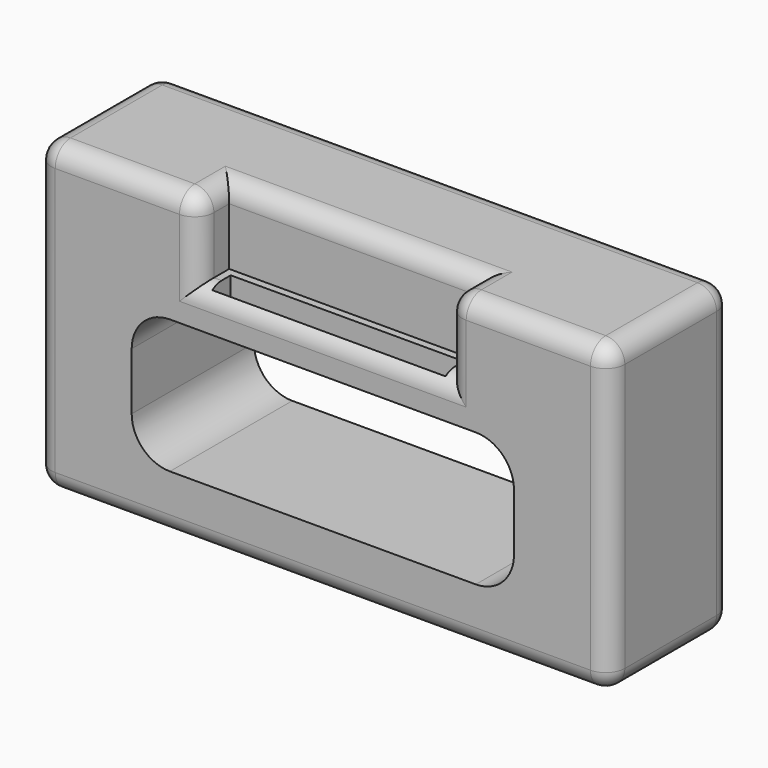
from build123d import *

# Parameters (mm, degrees)
F0_W          = 150
F0_H          = 40
F1_DEPTH      = 80
F2_W          = 65
F2_H          = 20
F3_DEPTH      = 10
F5_DEPTH      = 287
F6_W          = 61
F6_H          = 6
F7_DEPTH      = 25
F8_T1_DEPTH   = 65
F8_T3_DEPTH   = 70
F8_T5_DEPTH   = 32.5
F8_T7_DEPTH   = 32.5
F8_T9_DEPTH   = 30
F8_T11_DEPTH  = 140
F8_T13_DEPTH  = 15
F8_T15_DEPTH  = 5
F8_S19_W      = 5
F8_S19_H      = 5
F8_T20_DEPTH  = 5
F8_S25_W      = 5
F8_S25_H      = 5
F8_T26_DEPTH  = 5
F8_S31_W      = 5
F8_S31_H      = 5
F8_T32_DEPTH  = 5
F8_S37_W      = 5
F8_S37_H      = 5
F8_T38_DEPTH  = 5
F8_S43_W      = 5
F8_S43_H      = 5
F8_T44_DEPTH  = 5
F8_S49_W      = 5
F8_S49_H      = 5
F8_T50_DEPTH  = 5
F8_S55_W      = 5
F8_S55_H      = 5
F8_T56_DEPTH  = 5
F8_S61_W      = 5
F8_S61_H      = 5
F8_T62_DEPTH  = 5
F8_S67_W      = 5
F8_S67_H      = 5
F8_T68_DEPTH  = 5
F8_S73_W      = 5
F8_S73_H      = 5
F8_T74_DEPTH  = 5
F8_T81_DEPTH  = 17.5
F8_T85_DEPTH  = 77.5
F8_T92_DEPTH  = 77.5
F8_T96_DEPTH  = 17.5
F8_T103_DEPTH = 27.5
F8_T107_DEPTH = 77.5
F8_T114_DEPTH = 27.5
F8_T118_DEPTH = 77.5


# Not quite as in the source:
# - a fillet or chamfer that OpenCascade refuses, or shapes differently, is made with other operations: its cross-section is extruded or revolved along the edge and cut away or added


with BuildPart() as f1:
    # F0 (on Top) → F1 (new body)
    with BuildSketch(Plane.XY):
        with Locations((-14.0948228538, -1.1422424763)):
            Rectangle(F0_W, F0_H)
    extrude(amount=F1_DEPTH)

    # F2 (on face) → F3 (cut)
    with BuildSketch(Plane.XZ.offset(21.1422424763)):
        with Locations((-14.0948228538, 70)):
            Rectangle(F2_W, F2_H)
    extrude(amount=-F3_DEPTH, mode=Mode.SUBTRACT)

    # F4 (on face) → F5 (cut)
    with BuildSketch(Plane.XZ.offset(21.1422424763)):
        with BuildLine():
            Line((25.9051771462, 50), (-54.0948228538, 50))
            ThreePointArc((-54.0948228538, 50), (-61.1658906657, 47.0710678119), (-64.0948228538, 40))
            Line((-64.0948228538, 40), (-64.0948228538, 25))
            ThreePointArc((-64.0948228538, 25), (-61.1658906657, 17.9289321881), (-54.0948228538, 15))
            Line((-54.0948228538, 15), (25.9051771462, 15))
            ThreePointArc((25.9051771462, 15), (32.9762449581, 17.9289321881), (35.9051771462, 25))
            Line((35.9051771462, 25), (35.9051771462, 40))
            ThreePointArc((35.9051771462, 40), (32.9762449581, 47.0710678119), (25.9051771462, 50))
        make_face()
    extrude(amount=-F5_DEPTH, mode=Mode.SUBTRACT)

    # F6 (on face) → F7 (cut)
    with BuildSketch(Plane.XY.offset(60)):
        with Locations((-14.0948228538, -16.1422424763)):
            Rectangle(F6_W, F6_H)
    extrude(amount=-F7_DEPTH, mode=Mode.SUBTRACT)

    # F8: fillet of radius 5 on 19 edges, made by hand

    # F8_s2 → F8_t1 (cut)
    with BuildSketch(Plane.YZ.offset(-46.5948228538)):
        with BuildLine():
            ThreePointArc((-6.1422424763, 80), (-9.6777763823, 78.5355339059), (-11.1422424763, 75))
            Line((-11.1422424763, 75), (-11.1422424763, 80))
            Line((-11.1422424763, 80), (-6.1422424763, 80))
        make_face()
        with BuildLine():
            ThreePointArc((-21.1422424763, 55), (-19.6777763823, 58.5355339059), (-16.1422424763, 60))
            Line((-16.1422424763, 60), (-21.1422424763, 60))
            Line((-21.1422424763, 60), (-21.1422424763, 55))
        make_face()
    extrude(amount=F8_T1_DEPTH, mode=Mode.SUBTRACT)

    # F8_s4 → F8_t3 (cut)
    with BuildSketch(Plane.XY.offset(5)):
        with BuildLine():
            ThreePointArc((-84.0948228538, -21.1422424763), (-87.6303567597, -19.6777763823), (-89.0948228538, -16.1422424763))
            Line((-89.0948228538, -16.1422424763), (-89.0948228538, -21.1422424763))
            Line((-89.0948228538, -21.1422424763), (-84.0948228538, -21.1422424763))
        make_face()
        with BuildLine():
            ThreePointArc((60.9051771462, -16.1422424763), (59.4407110521, -19.6777763823), (55.9051771462, -21.1422424763))
            Line((55.9051771462, -21.1422424763), (60.9051771462, -21.1422424763))
            Line((60.9051771462, -21.1422424763), (60.9051771462, -16.1422424763))
        make_face()
        with BuildLine():
            ThreePointArc((-84.0948228538, 18.8577575237), (-87.6303567597, 17.3932914296), (-89.0948228538, 13.8577575237))
            Line((-89.0948228538, 13.8577575237), (-89.0948228538, 18.8577575237))
            Line((-89.0948228538, 18.8577575237), (-84.0948228538, 18.8577575237))
        make_face()
        with BuildLine():
            ThreePointArc((60.9051771462, 13.8577575237), (59.4407110521, 17.3932914296), (55.9051771462, 18.8577575237))
            Line((55.9051771462, 18.8577575237), (60.9051771462, 18.8577575237))
            Line((60.9051771462, 18.8577575237), (60.9051771462, 13.8577575237))
        make_face()
    extrude(amount=F8_T3_DEPTH, mode=Mode.SUBTRACT)

    # F8_s6 → F8_t5 (cut)
    with BuildSketch(Plane.YZ.offset(23.4051771462)):
        with BuildLine():
            ThreePointArc((-21.1422424763, 75), (-19.6777763823, 78.5355339059), (-16.1422424763, 80))
            Line((-16.1422424763, 80), (-21.1422424763, 80))
            Line((-21.1422424763, 80), (-21.1422424763, 75))
        make_face()
    extrude(amount=F8_T5_DEPTH, mode=Mode.SUBTRACT)

    # F8_s8 → F8_t7 (cut)
    with BuildSketch(Plane.YZ.offset(-84.0948228538)):
        with BuildLine():
            ThreePointArc((-21.1422424763, 75), (-19.6777763823, 78.5355339059), (-16.1422424763, 80))
            Line((-16.1422424763, 80), (-21.1422424763, 80))
            Line((-21.1422424763, 80), (-21.1422424763, 75))
        make_face()
    extrude(amount=F8_T7_DEPTH, mode=Mode.SUBTRACT)

    # F8_s10 → F8_t9 (cut)
    with BuildSketch(Plane.XZ.offset(-13.8577575237)):
        with BuildLine():
            ThreePointArc((60.9051771462, 5), (59.4407110521, 1.4644660941), (55.9051771462, 0))
            Line((55.9051771462, 0), (60.9051771462, 0))
            Line((60.9051771462, 0), (60.9051771462, 5))
        make_face()
        with BuildLine():
            ThreePointArc((-84.0948228538, 0), (-87.6303567597, 1.4644660941), (-89.0948228538, 5))
            Line((-89.0948228538, 5), (-89.0948228538, 0))
            Line((-89.0948228538, 0), (-84.0948228538, 0))
        make_face()
        with BuildLine():
            ThreePointArc((-84.0948228538, 80), (-87.6303567597, 78.5355339059), (-89.0948228538, 75))
            Line((-89.0948228538, 75), (-89.0948228538, 80))
            Line((-89.0948228538, 80), (-84.0948228538, 80))
        make_face()
        with BuildLine():
            ThreePointArc((60.9051771462, 75), (59.4407110521, 78.5355339059), (55.9051771462, 80))
            Line((55.9051771462, 80), (60.9051771462, 80))
            Line((60.9051771462, 80), (60.9051771462, 75))
        make_face()
    extrude(amount=F8_T9_DEPTH, mode=Mode.SUBTRACT)

    # F8_s12 → F8_t11 (cut)
    with BuildSketch(Plane.YZ.offset(-84.0948228538)):
        with BuildLine():
            ThreePointArc((18.8577575237, 5), (17.3932914296, 1.4644660941), (13.8577575237, 0))
            Line((13.8577575237, 0), (18.8577575237, 0))
            Line((18.8577575237, 0), (18.8577575237, 5))
        make_face()
        with BuildLine():
            ThreePointArc((-21.1422424763, 5), (-19.6777763823, 1.4644660941), (-16.1422424763, 0))
            Line((-16.1422424763, 0), (-21.1422424763, 0))
            Line((-21.1422424763, 0), (-21.1422424763, 5))
        make_face()
        with BuildLine():
            ThreePointArc((18.8577575237, 75), (17.3932914296, 78.5355339059), (13.8577575237, 80))
            Line((13.8577575237, 80), (18.8577575237, 80))
            Line((18.8577575237, 80), (18.8577575237, 75))
        make_face()
    extrude(amount=F8_T11_DEPTH, mode=Mode.SUBTRACT)

    # F8_s14 → F8_t13 (cut)
    with BuildSketch(Plane.XY.offset(60)):
        with BuildLine():
            ThreePointArc((-51.5948228538, -21.1422424763), (-48.0592889479, -19.6777763823), (-46.5948228538, -16.1422424763))
            Line((-46.5948228538, -16.1422424763), (-46.5948228538, -21.1422424763))
            Line((-46.5948228538, -21.1422424763), (-51.5948228538, -21.1422424763))
        make_face()
        with BuildLine():
            ThreePointArc((23.4051771462, -21.1422424763), (19.8696432403, -19.6777763823), (18.4051771462, -16.1422424763))
            Line((18.4051771462, -16.1422424763), (18.4051771462, -21.1422424763))
            Line((18.4051771462, -21.1422424763), (23.4051771462, -21.1422424763))
        make_face()
    extrude(amount=F8_T13_DEPTH, mode=Mode.SUBTRACT)

    # F8_s16 → F8_t15 (cut)
    with BuildSketch(Plane.XZ.offset(11.1422424763)):
        with BuildLine():
            ThreePointArc((-51.5948228538, 80), (-48.0592889479, 78.5355339059), (-46.5948228538, 75))
            Line((-46.5948228538, 75), (-46.5948228538, 80))
            Line((-46.5948228538, 80), (-51.5948228538, 80))
        make_face()
        with BuildLine():
            ThreePointArc((23.4051771462, 80), (19.8696432403, 78.5355339059), (18.4051771462, 75))
            Line((18.4051771462, 75), (18.4051771462, 80))
            Line((18.4051771462, 80), (23.4051771462, 80))
        make_face()
    extrude(amount=F8_T15_DEPTH, mode=Mode.SUBTRACT)


with BuildPart() as f8_tool18:
    # F8_s19 → F8_t20 (new body)
    with BuildSketch(Plane.XZ.offset(16.1422424763)):
        with Locations((-86.5948228538, 2.5)):
            Rectangle(F8_S19_W, F8_S19_H)
    extrude(amount=F8_T20_DEPTH)

    # F8_s21 → F8_t22 (revolve, cut)
    with BuildSketch(Plane(origin=(-84.0948228538, -16.1422424763, 5), x_dir=(0.7071067812, 0, 0.7071067812), z_dir=(0.7071067812, 0, -0.7071067812))):
        with BuildLine():
            ThreePointArc((0, -5), (5, 0), (0, 5))
            Line((0, 5), (0, -5))
        make_face()
    revolve(axis=Axis((-84.0948228538, -16.1422424763, 5), (0, -1, 0)), mode=Mode.SUBTRACT)


with BuildPart() as f1_1:
    add(f1.part)

    # F8_t17: cut F8_tool18
    add(f8_tool18.part, mode=Mode.SUBTRACT)


with BuildPart() as f8_tool24:
    # F8_s25 → F8_t26 (new body)
    with BuildSketch(Plane.XZ.offset(16.1422424763)):
        with Locations((-86.5948228538, 77.5)):
            Rectangle(F8_S25_W, F8_S25_H)
    extrude(amount=F8_T26_DEPTH)

    # F8_s27 → F8_t28 (revolve, cut)
    with BuildSketch(Plane(origin=(-84.0948228538, -16.1422424763, 75), x_dir=(0.7071067812, 0, -0.7071067812), z_dir=(-0.7071067812, 0, -0.7071067812))):
        with BuildLine():
            ThreePointArc((0, -5), (5, 0), (0, 5))
            Line((0, 5), (0, -5))
        make_face()
    revolve(axis=Axis((-84.0948228538, -16.1422424763, 75), (0, -1, 0)), mode=Mode.SUBTRACT)


with BuildPart() as f1_2:
    add(f1_1.part)

    # F8_t23: cut F8_tool24
    add(f8_tool24.part, mode=Mode.SUBTRACT)


with BuildPart() as f8_tool30:
    # F8_s31 → F8_t32 (new body)
    with BuildSketch(Plane.YZ.offset(55.9051771462)):
        with Locations((-18.6422424763, 2.5)):
            Rectangle(F8_S31_W, F8_S31_H)
    extrude(amount=F8_T32_DEPTH)

    # F8_s33 → F8_t34 (revolve, cut)
    with BuildSketch(Plane(origin=(55.9051771462, -16.1422424763, 5), x_dir=(0, 0.7071067812, 0.7071067812), z_dir=(0, 0.7071067812, -0.7071067812))):
        with BuildLine():
            ThreePointArc((0, -5), (5, 0), (0, 5))
            Line((0, 5), (0, -5))
        make_face()
    revolve(axis=Axis((55.9051771462, -16.1422424763, 5), (1, 0, 0)), mode=Mode.SUBTRACT)


with BuildPart() as f1_3:
    add(f1_2.part)

    # F8_t29: cut F8_tool30
    add(f8_tool30.part, mode=Mode.SUBTRACT)


with BuildPart() as f8_tool36:
    # F8_s37 → F8_t38 (new body)
    with BuildSketch(Plane.YZ.offset(55.9051771462)):
        with Locations((-18.6422424763, 77.5)):
            Rectangle(F8_S37_W, F8_S37_H)
    extrude(amount=F8_T38_DEPTH)

    # F8_s39 → F8_t40 (revolve, cut)
    with BuildSketch(Plane(origin=(55.9051771462, -16.1422424763, 75), x_dir=(0, 0.7071067812, -0.7071067812), z_dir=(0, -0.7071067812, -0.7071067812))):
        with BuildLine():
            ThreePointArc((0, -5), (5, 0), (0, 5))
            Line((0, 5), (0, -5))
        make_face()
    revolve(axis=Axis((55.9051771462, -16.1422424763, 75), (1, 0, 0)), mode=Mode.SUBTRACT)


with BuildPart() as f1_4:
    add(f1_3.part)

    # F8_t35: cut F8_tool36
    add(f8_tool36.part, mode=Mode.SUBTRACT)


with BuildPart() as f8_tool42:
    # F8_s43 → F8_t44 (new body)
    with BuildSketch(Plane.XZ.offset(16.1422424763)):
        with Locations((20.9051771462, 77.5)):
            Rectangle(F8_S43_W, F8_S43_H)
    extrude(amount=F8_T44_DEPTH)

    # F8_s45 → F8_t46 (revolve, cut)
    with BuildSketch(Plane(origin=(23.4051771462, -16.1422424763, 75), x_dir=(0.7071067812, 0, -0.7071067812), z_dir=(-0.7071067812, 0, -0.7071067812))):
        with BuildLine():
            ThreePointArc((0, -5), (5, 0), (0, 5))
            Line((0, 5), (0, -5))
        make_face()
    revolve(axis=Axis((23.4051771462, -16.1422424763, 75), (0, -1, 0)), mode=Mode.SUBTRACT)


with BuildPart() as f1_5:
    add(f1_4.part)

    # F8_t41: cut F8_tool42
    add(f8_tool42.part, mode=Mode.SUBTRACT)


with BuildPart() as f8_tool48:
    # F8_s49 → F8_t50 (new body)
    with BuildSketch(Plane.XZ.offset(16.1422424763)):
        with Locations((-49.0948228538, 77.5)):
            Rectangle(F8_S49_W, F8_S49_H)
    extrude(amount=F8_T50_DEPTH)

    # F8_s51 → F8_t52 (revolve, cut)
    with BuildSketch(Plane(origin=(-51.5948228538, -16.1422424763, 75), x_dir=(-0.7071067812, 0, -0.7071067812), z_dir=(-0.7071067812, 0, 0.7071067812))):
        with BuildLine():
            ThreePointArc((0, -5), (5, 0), (0, 5))
            Line((0, 5), (0, -5))
        make_face()
    revolve(axis=Axis((-51.5948228538, -16.1422424763, 75), (0, -1, 0)), mode=Mode.SUBTRACT)


with BuildPart() as f1_6:
    add(f1_5.part)

    # F8_t47: cut F8_tool48
    add(f8_tool48.part, mode=Mode.SUBTRACT)


with BuildPart() as f8_tool54:
    # F8_s55 → F8_t56 (new body)
    with BuildSketch(Plane.YZ.offset(55.9051771462)):
        with Locations((16.3577575237, 2.5)):
            Rectangle(F8_S55_W, F8_S55_H)
    extrude(amount=F8_T56_DEPTH)

    # F8_s57 → F8_t58 (revolve, cut)
    with BuildSketch(Plane(origin=(55.9051771462, 13.8577575237, 5), x_dir=(0, -0.7071067812, 0.7071067812), z_dir=(0, 0.7071067812, 0.7071067812))):
        with BuildLine():
            ThreePointArc((0, -5), (5, 0), (0, 5))
            Line((0, 5), (0, -5))
        make_face()
    revolve(axis=Axis((55.9051771462, 13.8577575237, 5), (1, 0, 0)), mode=Mode.SUBTRACT)


with BuildPart() as f1_7:
    add(f1_6.part)

    # F8_t53: cut F8_tool54
    add(f8_tool54.part, mode=Mode.SUBTRACT)


with BuildPart() as f8_tool60:
    # F8_s61 → F8_t62 (new body)
    with BuildSketch(Plane.XZ.offset(-13.8577575237)):
        with Locations((-86.5948228538, 2.5)):
            Rectangle(F8_S61_W, F8_S61_H)
    extrude(amount=-F8_T62_DEPTH)

    # F8_s63 → F8_t64 (revolve, cut)
    with BuildSketch(Plane(origin=(-84.0948228538, 13.8577575237, 5), x_dir=(0.7071067812, 0, 0.7071067812), z_dir=(-0.7071067812, 0, 0.7071067812))):
        with BuildLine():
            ThreePointArc((0, -5), (5, 0), (0, 5))
            Line((0, 5), (0, -5))
        make_face()
    revolve(axis=Axis((-84.0948228538, 13.8577575237, 5), (0, 1, 0)), mode=Mode.SUBTRACT)


with BuildPart() as f1_8:
    add(f1_7.part)

    # F8_t59: cut F8_tool60
    add(f8_tool60.part, mode=Mode.SUBTRACT)


with BuildPart() as f8_tool66:
    # F8_s67 → F8_t68 (new body)
    with BuildSketch(Plane.XZ.offset(-13.8577575237)):
        with Locations((-86.5948228538, 77.5)):
            Rectangle(F8_S67_W, F8_S67_H)
    extrude(amount=-F8_T68_DEPTH)

    # F8_s69 → F8_t70 (revolve, cut)
    with BuildSketch(Plane(origin=(-84.0948228538, 13.8577575237, 75), x_dir=(0.7071067812, 0, -0.7071067812), z_dir=(0.7071067812, 0, 0.7071067812))):
        with BuildLine():
            ThreePointArc((0, -5), (5, 0), (0, 5))
            Line((0, 5), (0, -5))
        make_face()
    revolve(axis=Axis((-84.0948228538, 13.8577575237, 75), (0, 1, 0)), mode=Mode.SUBTRACT)


with BuildPart() as f1_9:
    add(f1_8.part)

    # F8_t65: cut F8_tool66
    add(f8_tool66.part, mode=Mode.SUBTRACT)


with BuildPart() as f8_tool72:
    # F8_s73 → F8_t74 (new body)
    with BuildSketch(Plane.YZ.offset(55.9051771462)):
        with Locations((16.3577575237, 77.5)):
            Rectangle(F8_S73_W, F8_S73_H)
    extrude(amount=F8_T74_DEPTH)

    # F8_s75 → F8_t76 (revolve, cut)
    with BuildSketch(Plane(origin=(55.9051771462, 13.8577575237, 75), x_dir=(0, -0.7071067812, -0.7071067812), z_dir=(0, -0.7071067812, 0.7071067812))):
        with BuildLine():
            ThreePointArc((0, -5), (5, 0), (0, 5))
            Line((0, 5), (0, -5))
        make_face()
    revolve(axis=Axis((55.9051771462, 13.8577575237, 75), (1, 0, 0)), mode=Mode.SUBTRACT)


with BuildPart() as f1_10:
    add(f1_9.part)

    # F8_t71: cut F8_tool72
    add(f8_tool72.part, mode=Mode.SUBTRACT)


with BuildPart() as f8_tool79:
    # F8_s80 → F8_t81 (new body)
    with BuildSketch(Plane.XZ.offset(16.1422424763)):
        with BuildLine():
            ThreePointArc((23.4051771462, 80), (19.8696432403, 78.5355339059), (18.4051771462, 75))
            Line((18.4051771462, 75), (18.4051771462, 80))
            Line((18.4051771462, 80), (23.4051771462, 80))
        make_face()
    extrude(amount=-F8_T81_DEPTH)

    split(bisect_by=Plane.XZ.offset(11.1422424763), keep=Keep.BOTTOM)


with BuildPart() as f8_tool83:
    # F8_s84 → F8_t85 (new body)
    with BuildSketch(Plane.YZ.offset(30.9051771462)):
        with BuildLine():
            ThreePointArc((-6.1422424763, 80), (-9.6777763823, 78.5355339059), (-11.1422424763, 75))
            Line((-11.1422424763, 75), (-11.1422424763, 80))
            Line((-11.1422424763, 80), (-6.1422424763, 80))
        make_face()
    extrude(amount=-F8_T85_DEPTH)

    split(bisect_by=Plane.YZ.offset(18.4051771462), keep=Keep.TOP)


with BuildPart() as f8_tool79_1:
    add(f8_tool79.part)

    # F8_t87: intersect F8_tool83
    add(f8_tool83.part, mode=Mode.INTERSECT)


with BuildPart() as f1_11:
    add(f1_10.part)

    # F8_t77: cut F8_tool79
    add(f8_tool79_1.part, mode=Mode.SUBTRACT)


with BuildPart() as f8_tool90:
    # F8_s91 → F8_t92 (new body)
    with BuildSketch(Plane.YZ.offset(18.4051771462)):
        with BuildLine():
            ThreePointArc((-6.1422424763, 80), (-9.6777763823, 78.5355339059), (-11.1422424763, 75))
            Line((-11.1422424763, 75), (-11.1422424763, 80))
            Line((-11.1422424763, 80), (-6.1422424763, 80))
        make_face()
    extrude(amount=-F8_T92_DEPTH)

    split(bisect_by=Plane.YZ.offset(-46.5948228538), keep=Keep.BOTTOM)


with BuildPart() as f8_tool94:
    # F8_s95 → F8_t96 (new body)
    with BuildSketch(Plane.XZ.offset(16.1422424763)):
        with BuildLine():
            ThreePointArc((-51.5948228538, 80), (-48.0592889479, 78.5355339059), (-46.5948228538, 75))
            Line((-46.5948228538, 75), (-46.5948228538, 80))
            Line((-46.5948228538, 80), (-51.5948228538, 80))
        make_face()
    extrude(amount=-F8_T96_DEPTH)

    split(bisect_by=Plane.XZ.offset(11.1422424763), keep=Keep.BOTTOM)


with BuildPart() as f8_tool90_1:
    add(f8_tool90.part)

    # F8_t98: intersect F8_tool94
    add(f8_tool94.part, mode=Mode.INTERSECT)


with BuildPart() as f1_12:
    add(f1_11.part)

    # F8_t88: cut F8_tool90
    add(f8_tool90_1.part, mode=Mode.SUBTRACT)


with BuildPart() as f8_tool101:
    # F8_s102 → F8_t103 (new body)
    with BuildSketch(Plane.XY.offset(75)):
        with BuildLine():
            ThreePointArc((-51.5948228538, -21.1422424763), (-48.0592889479, -19.6777763823), (-46.5948228538, -16.1422424763))
            Line((-46.5948228538, -16.1422424763), (-46.5948228538, -21.1422424763))
            Line((-46.5948228538, -21.1422424763), (-51.5948228538, -21.1422424763))
        make_face()
    extrude(amount=-F8_T103_DEPTH)

    split(bisect_by=Plane.XY.offset(60), keep=Keep.BOTTOM)


with BuildPart() as f8_tool105:
    # F8_s106 → F8_t107 (new body)
    with BuildSketch(Plane.YZ.offset(-59.0948228538)):
        with BuildLine():
            ThreePointArc((-21.1422424763, 55), (-19.6777763823, 58.5355339059), (-16.1422424763, 60))
            Line((-16.1422424763, 60), (-21.1422424763, 60))
            Line((-21.1422424763, 60), (-21.1422424763, 55))
        make_face()
    extrude(amount=F8_T107_DEPTH)

    split(bisect_by=Plane.YZ.offset(-46.5948228538), keep=Keep.BOTTOM)


with BuildPart() as f8_tool101_1:
    add(f8_tool101.part)

    # F8_t109: intersect F8_tool105
    add(f8_tool105.part, mode=Mode.INTERSECT)


with BuildPart() as f1_13:
    add(f1_12.part)

    # F8_t99: cut F8_tool101
    add(f8_tool101_1.part, mode=Mode.SUBTRACT)


with BuildPart() as f8_tool112:
    # F8_s113 → F8_t114 (new body)
    with BuildSketch(Plane.XY.offset(47.5)):
        with BuildLine():
            ThreePointArc((23.4051771462, -21.1422424763), (19.8696432403, -19.6777763823), (18.4051771462, -16.1422424763))
            Line((18.4051771462, -16.1422424763), (18.4051771462, -21.1422424763))
            Line((18.4051771462, -21.1422424763), (23.4051771462, -21.1422424763))
        make_face()
    extrude(amount=F8_T114_DEPTH)

    split(bisect_by=Plane.XY.offset(60), keep=Keep.BOTTOM)


with BuildPart() as f8_tool116:
    # F8_s117 → F8_t118 (new body)
    with BuildSketch(Plane.YZ.offset(-46.5948228538)):
        with BuildLine():
            ThreePointArc((-21.1422424763, 55), (-19.6777763823, 58.5355339059), (-16.1422424763, 60))
            Line((-16.1422424763, 60), (-21.1422424763, 60))
            Line((-21.1422424763, 60), (-21.1422424763, 55))
        make_face()
    extrude(amount=F8_T118_DEPTH)

    split(bisect_by=Plane.YZ.offset(18.4051771462), keep=Keep.TOP)


with BuildPart() as f8_tool112_1:
    add(f8_tool112.part)

    # F8_t120: intersect F8_tool116
    add(f8_tool116.part, mode=Mode.INTERSECT)


with BuildPart() as f1_14:
    add(f1_13.part)

    # F8_t110: cut F8_tool112
    add(f8_tool112_1.part, mode=Mode.SUBTRACT)


solid = f1_14.part
